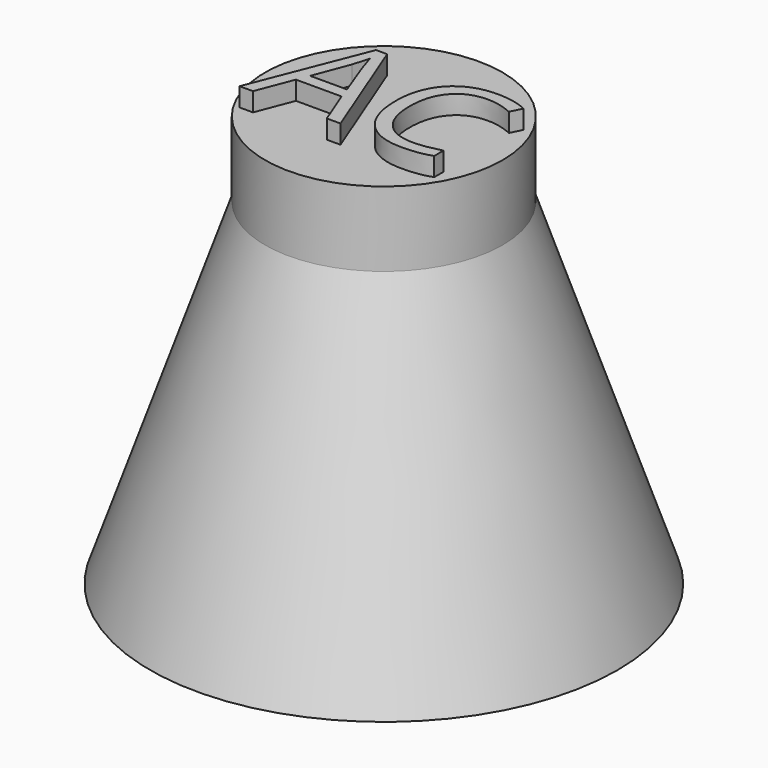
from build123d import *

# Parameters (mm, degrees)
F0_W         = 4.85
F0_H         = 4
F0_W_2       = 1.5
F2_TEXT_SIZE = 8.5267813928
F3_DEPTH     = 1


# Not quite as in the source:
# - Text() gives the source's letters only with a copy of the font that has no kerning and outlines rounded to 1/6400 em; it was checked with that copy


with BuildPart() as f1:
    # F0 (on Front) → F1 (revolve)
    with BuildSketch(Plane.XZ):
        with Locations((2.425, 20)):
            Rectangle(F0_W, F0_H)
        with Locations((5.6, 20)):
            Rectangle(F0_W_2, F0_H)
        Polygon((4.85, 18), (11, 0), (12.5, 0), (6.35, 18), align=None)
        Polygon((0, 18), (0, 0), (11, 0), (4.85, 18), align=None)
    revolve(axis=Axis((0, 0, 9), (0, 0, 1)))

    # F2 (on face) → F3 (join)
    with BuildSketch(Plane.XY.offset(22)):
        with Locations((-5.2024447359, -3.1394062098)):
            Text('AC', F2_TEXT_SIZE, font='Open Sans', text_align=(TextAlign.LEFT, TextAlign.BOTTOM))
    extrude(amount=F3_DEPTH)


solid = f1.part
